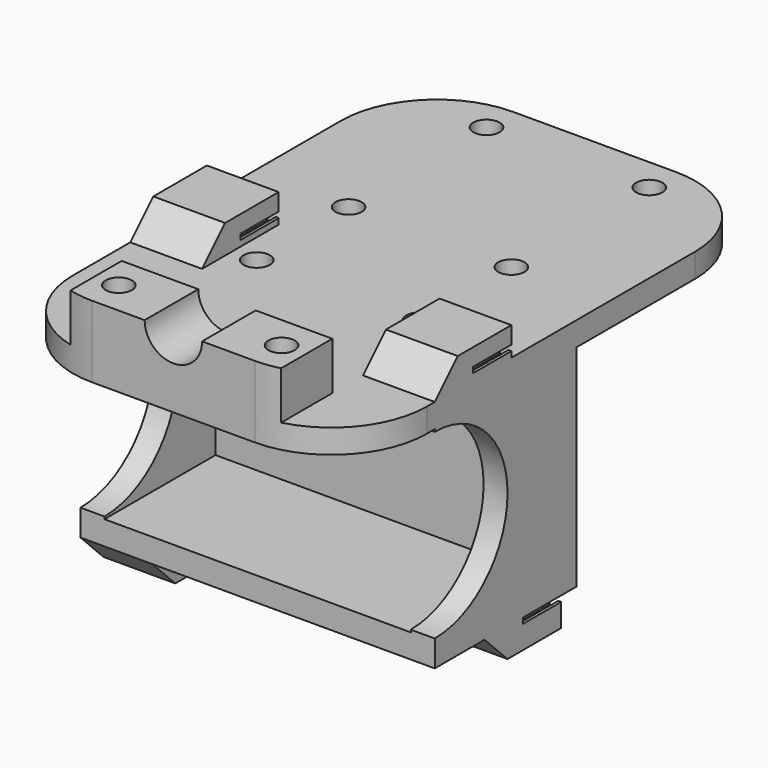
from build123d import *

# Parameters (mm, degrees)
F0_R      = 2.75
F1_DEPTH  = 5
F2_W      = 15
F2_H      = 20
F3_DEPTH  = 6
F4_DEPTH  = 5
F5_W      = 15
F5_H      = 20
F6_DEPTH  = 11
F8_W      = 44
F8_H      = 8
F9_DEPTH  = 39
F10_W     = 15
F10_H     = 20
F11_DEPTH = 11
F13_W     = 44
F13_H     = 37
F13_W_2   = 15
F14_DEPTH = 5
F15_DEPTH = 10
F16_W     = 15
F16_H     = 20
F17_DEPTH = 6
F18_DEPTH = 5
F20_DEPTH = 10
F21_SIZE  = 5.99999
F22_W     = 15
F22_H     = 13
F22_H_2   = 4
F22_H_3   = 17
F23_DEPTH = 5
F24_W     = 10
F24_H     = 8
F25_DEPTH = 39
F26_DEPTH = 10
F27_W     = 44
F27_H     = 14
F28_DEPTH = 10
F30_DEPTH = 14
F31_DEPTH = 15
F32_R     = 19
F33_DEPTH = 74
F35_DEPTH = 10
F36_W     = 15
F36_H     = 51
F36_H_2   = 22
F37_DEPTH = 5
F38_R     = 20


# Not quite as in the source:
# - a fillet or chamfer is up to 0.001 mm smaller than in the source, because OpenCascade refuses the exact size


with BuildPart() as f1:
    # F0 (on Top) → F1 (new body)
    with BuildSketch(Plane.XY):
        Polygon((0, 55), (-22, 55), (-22, -55), (0, -55), (22, -55), (22, 55), align=None)
        with Locations((-17, -48)):
            Circle(F0_R, mode=Mode.SUBTRACT)
        with Locations((-17, -12)):
            Circle(F0_R, mode=Mode.SUBTRACT)
        with Locations((17, -48)):
            Circle(F0_R, mode=Mode.SUBTRACT)
        with Locations((17, -12)):
            Circle(F0_R, mode=Mode.SUBTRACT)
        with Locations((-17, 12)):
            Circle(F0_R, mode=Mode.SUBTRACT)
        with Locations((-17, 48)):
            Circle(F0_R, mode=Mode.SUBTRACT)
        with Locations((17, 12)):
            Circle(F0_R, mode=Mode.SUBTRACT)
        with Locations((17, 48)):
            Circle(F0_R, mode=Mode.SUBTRACT)
    extrude(amount=F1_DEPTH)



with BuildPart() as f3:
    # F2 (on face) → F3 (new body)
    with BuildSketch(Plane.XY.offset(5)):
        with Locations((29.5, -23)):
            Rectangle(F2_W, F2_H)
    extrude(amount=F3_DEPTH)


with BuildPart() as f1_1:
    add(f1.part)
    # F4 (add): a face of the model
    f4_faces = [f3.part.faces().sort_by_distance(p)[0] for p in [
        (29.5, -23, 5),
    ]]

    add(f3.part)  # F4 merges F3
    extrude(f4_faces, amount=F4_DEPTH)

    # F5 (on Top) → F6 (join)
    with BuildSketch(Plane.XY):
        with Locations((-29.5, -10)):
            Rectangle(F5_W, F5_H)
    extrude(amount=F6_DEPTH)

    # F8 (on face) → F9 (join)
    with BuildSketch(Plane.XY):
        Rectangle(F8_W, F8_H)
    extrude(amount=-F9_DEPTH)

    # F10 (on face) → F11 (join)
    with BuildSketch(Plane(origin=(0, 0, -39), x_dir=(1, 0, 0), z_dir=(0, 0, -1))):
        with Locations((29.5, 10)):
            Rectangle(F10_W, F10_H)
    extrude(amount=F11_DEPTH)

    # F13 (on face) → F14 (join)
    with BuildSketch(Plane(origin=(0, 0, -39), x_dir=(1, 0, 0), z_dir=(0, 0, -1))):
        with Locations((0, 14.5)):
            Rectangle(F13_W, F13_H)
        with Locations((29.5, 14.5)):
            Rectangle(F13_W_2, F13_H)
        with Locations((-29.5, 14.5)):
            Rectangle(F13_W_2, F13_H)
    extrude(amount=F14_DEPTH)

    # F12 (on face) → F15 (cut)
    with BuildSketch(Plane(origin=(0, 0, 0), x_dir=(-1, 0, 0), z_dir=(0, 1, 0))):
        Polygon((-36.39, -45.18), (-36.39, -46.4), (-34.61, -46.4), (-34.61, -45.18), (-33.39, -45.18), (-33.39, -46.4), (-31.61, -46.4), (-31.61, -45.18), (-30.39, -45.18), (-30.39, -46.4), (-28.61, -46.4), (-28.61, -45.18), (-27.39, -45.18), (-27.39, -46.4), (-25.61, -46.4), (-25.61, -45.18), (-24.39, -45.18), (-24.39, -46.4), (-22.61, -46.4), (-22.61, -45.18), (-22, -45.18), (-22, -44), (-37, -44), (-37, -45.18), align=None)
    extrude(amount=-F15_DEPTH, mode=Mode.SUBTRACT)



with BuildPart() as f17:
    # F16 (on face) → F17 (new body)
    with BuildSketch(Plane(origin=(0, 0, -44), x_dir=(1, 0, 0), z_dir=(0, 0, -1))):
        with Locations((-29.5, 23)):
            Rectangle(F16_W, F16_H)
    extrude(amount=F17_DEPTH)


with BuildPart() as f1_2:
    add(f1_1.part)
    # F18 (add): a face of the model
    f18_faces = [f17.part.faces().sort_by_distance(p)[0] for p in [
        (-29.5, -23, -44),
    ]]

    add(f17.part)  # F18 merges F17
    extrude(f18_faces, amount=F18_DEPTH)

    # F19 (on face) → F20 (cut)
    with BuildSketch(Plane(origin=(0, -13, 0), x_dir=(-1, 0, 0), z_dir=(0, 1, 0))):
        Polygon((22.61, -45.18), (22.61, -46.4), (24.39, -46.4), (24.39, -45.18), (25.61, -45.18), (25.61, -46.4), (27.39, -46.4), (27.39, -45.18), (28.61, -45.18), (28.61, -46.4), (30.39, -46.4), (30.39, -45.18), (31.61, -45.18), (31.61, -46.4), (33.39, -46.4), (33.39, -45.18), (34.61, -45.18), (34.61, -46.4), (36.39, -46.4), (36.39, -45.18), (37, -45.18), (37, -44), (22, -44), (22, -45.18), align=None)
    extrude(amount=-F20_DEPTH, mode=Mode.SUBTRACT)

    # F21 (size 6 in the source; OpenCascade refuses exactly that, so slightly less here)
    f21_edges = [f1_2.edges().sort_by_distance(p)[0] for p in [
        (-29.5, -20, 11),
        (29.5, -33, 11),
        (29.5, -20, -50),
        (-29.5, -33, -50),
    ]]
    chamfer(f21_edges, length=F21_SIZE)

    # F22 (on Top) → F23 (join)
    with BuildSketch(Plane.XY):
        with Locations((-29.5, -26.5)):
            Rectangle(F22_W, F22_H)
        with Locations((-29.5, 2)):
            Rectangle(F22_W, F22_H_2)
        with Locations((29.5, -4.5)):
            Rectangle(F22_W, F22_H_3)
    extrude(amount=F23_DEPTH)

    # F24 (on face) → F25 (join)
    with BuildSketch(Plane(origin=(0, 0, 0), x_dir=(1, 0, 0), z_dir=(0, 0, -1))):
        Polygon((32, -4), (37, -4), (37, 33), (32, 33), (32, 4), align=None)
        with Locations((27, 0)):
            Rectangle(F24_W, F24_H)
        Polygon((-37, 33), (-37, -4), (-32, -4), (-32, 4), (-32, 33), align=None)
        with Locations((-27, 0)):
            Rectangle(F24_W, F24_H)
    extrude(amount=F25_DEPTH)

    # F7 (on face) → F26 (cut)
    with BuildSketch(Plane(origin=(0, 0, 0), x_dir=(-1, 0, 0), z_dir=(0, 1, 0))):
        Polygon((22.61, 6.22), (22.61, 5), (24.39, 5), (24.39, 6.22), (25.61, 6.22), (25.61, 5), (27.39, 5), (27.39, 6.22), (28.61, 6.22), (28.61, 5), (30.39, 5), (30.39, 6.22), (31.61, 6.22), (31.61, 5), (33.39, 5), (33.39, 6.22), (34.61, 6.22), (34.61, 5), (36.39, 5), (36.39, 6.22), (37, 6.22), (37, 7.4), (22, 7.4), (22, 6.22), align=None)
    extrude(amount=-F26_DEPTH, mode=Mode.SUBTRACT)

    # F27 (on face) → F28 (join)
    with BuildSketch(Plane.XY.offset(5)):
        with Locations((0, -48)):
            Rectangle(F27_W, F27_H)
    extrude(amount=F28_DEPTH)

    # F29 (on face) → F30 (cut)
    with BuildSketch(Plane(origin=(0, -41, 0), x_dir=(-1, 0, 0), z_dir=(0, 1, 0))):
        with BuildLine():
            Line((-6, 15), (6, 15))
            ThreePointArc((6, 15), (0, 21), (-6, 15))
        make_face()
        with BuildLine():
            ThreePointArc((-6, 15), (0, 9), (6, 15))
            Line((6, 15), (-6, 15))
        make_face()
    extrude(amount=-F30_DEPTH, mode=Mode.SUBTRACT)

    # F0 (on Top) → F31 (cut)
    with BuildSketch(Plane.XY):
        with Locations((-17, -48)):
            Circle(F0_R)
        with Locations((17, -48)):
            Circle(F0_R)
    extrude(amount=F31_DEPTH, mode=Mode.SUBTRACT)

    # F32 (on face) → F33 (cut)
    with BuildSketch(Plane.YZ.offset(37)):
        with Locations((-33, -19.5)):
            Circle(F32_R)
    extrude(amount=-F33_DEPTH, mode=Mode.SUBTRACT)

    # F34 (on face) → F35 (cut)
    with BuildSketch(Plane(origin=(0, -13, 0), x_dir=(-1, 0, 0), z_dir=(0, 1, 0))):
        Polygon((-36.39, 6.22), (-36.39, 5), (-34.61, 5), (-34.61, 6.22), (-33.39, 6.22), (-33.39, 5), (-31.61, 5), (-31.61, 6.22), (-30.39, 6.22), (-30.39, 5), (-28.61, 5), (-28.61, 6.22), (-27.39, 6.22), (-27.39, 5), (-25.61, 5), (-25.61, 6.22), (-24.39, 6.22), (-24.39, 5), (-22.61, 5), (-22.61, 6.22), (-22, 6.22), (-22, 7.4), (-37, 7.4), (-37, 6.22), align=None)
    extrude(amount=-F35_DEPTH, mode=Mode.SUBTRACT)

    # F36 (on Top) → F37 (join)
    with BuildSketch(Plane.XY):
        with Locations((-29.5, 29.5)):
            Rectangle(F36_W, F36_H)
        with Locations((29.5, 29.5)):
            Rectangle(F36_W, F36_H)
        with Locations((-29.5, -44)):
            Rectangle(F36_W, F36_H_2)
        with Locations((29.5, -44)):
            Rectangle(F36_W, F36_H_2)
    extrude(amount=F37_DEPTH)

    # F38
    f38_edges = [f1_2.edges().sort_by_distance(p)[0] for p in [
        (-37, -55, 2.5),
        (37, -55, 2.5),
        (37, 55, 2.5),
        (-37, 55, 2.5),
    ]]
    fillet(f38_edges, radius=F38_R)


solid = f1_2.part
